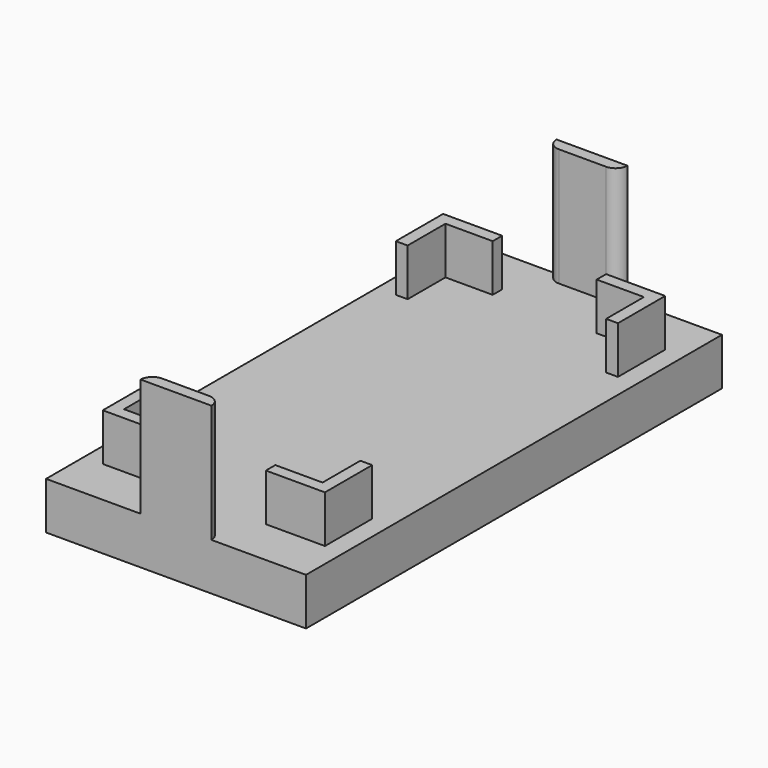
from build123d import *

# Parameters (mm, degrees)
F0_W     = 110
F0_H     = 220
F1_DEPTH = 20
F3_DEPTH = 20
F4_W     = 30
F4_H     = 5
F5_DEPTH = 50
F6_R     = 4.99999


# Not quite as in the source:
# - a fillet or chamfer is up to 0.001 mm smaller than in the source, because OpenCascade refuses the exact size


with BuildPart() as f1:
    # F0 (on Top) → F1 (new body)
    with BuildSketch(Plane.XY):
        with Locations((55, -110)):
            Rectangle(F0_W, F0_H)
    extrude(amount=F1_DEPTH)

    # F2 (on face) → F3 (join)
    with BuildSketch(Plane.XY.offset(20)):
        Polygon((8, -20), (8, -45), (13, -45), (13, -25), (33, -25), (33, -20), align=None)
        Polygon((77, -20), (77, -25), (97, -25), (97, -45), (102, -45), (102, -20), align=None)
        Polygon((33, -200), (33, -195), (13, -195), (13, -175), (8, -175), (8, -200), align=None)
        Polygon((97, -175), (97, -195), (77, -195), (77, -200), (102, -200), (102, -175), align=None)
    extrude(amount=F3_DEPTH)

    # F4 (on face) → F5 (join)
    with BuildSketch(Plane.XY.offset(20)):
        with Locations((55, -2.5)):
            Rectangle(F4_W, F4_H)
        with Locations((55, -217.5)):
            Rectangle(F4_W, F4_H)
    extrude(amount=F5_DEPTH)

    # F6 (radius 5 in the source; OpenCascade refuses exactly that, so slightly less here)
    f6_edges = [f1.edges().sort_by_distance(p)[0] for p in [
        (40, -5, 45),
        (70, -5, 45),
        (40, -215, 45),
        (70, -215, 45),
    ]]
    fillet(f6_edges, radius=F6_R)


solid = f1.part
